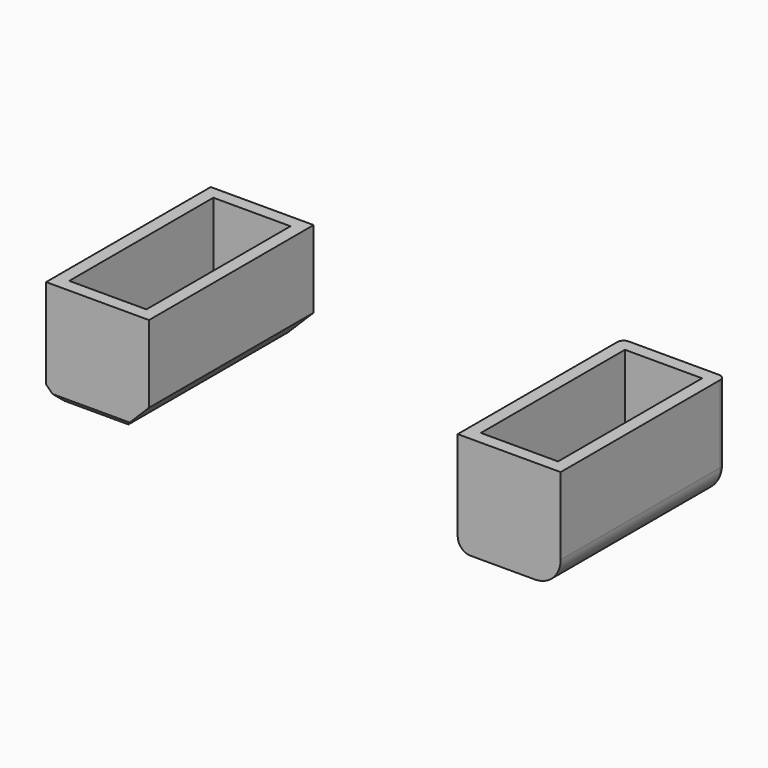
from build123d import *

# Parameters (mm, degrees)
F0_W     = 12.7
F0_H     = 25.4
F1_DEPTH = 12.7
F3_SIZE  = 3.175
F4_SIZE  = 1.5875
F5_SIZE  = 0.79375
F6_T     = -1.5875
F7_R     = 3.175
F8_R     = 1.5875
F9_R     = 0.79375
F10_T    = 1.5875


# Not quite as in the source:
# - a shell that OpenCascade refuses in one call is made with other operations: the cavity is built on its own and cut out


with BuildPart() as f1:
    # F0 (on Top) → F1 (new body)
    with BuildSketch(Plane.XY):
        with Locations((-17.8713803947, 23.258962822)):
            Rectangle(F0_W, F0_H)
    extrude(amount=F1_DEPTH)


with BuildPart() as f2_1:
    # F2: copy of F1
    add(f1.part.moved(Location((50.8, 0, 0))))

    # F7
    f7_edges = [f2_1.edges().sort_by_distance(p)[0] for p in [
        (39.27862, 23.258963, 0),
    ]]
    fillet(f7_edges, radius=F7_R)

    # F8
    f8_edges = [f2_1.edges().sort_by_distance(p)[0] for p in [
        (26.57862, 23.258963, 0),
    ]]
    fillet(f8_edges, radius=F8_R)

    # F9
    f9_edges = [f2_1.edges().sort_by_distance(p)[0] for p in [
        (32.13487, 35.958963, 0),
    ]]
    fillet(f9_edges, radius=F9_R)

    # F10: shell of thickness 1.5875, made by hand


with BuildPart() as f1_1:
    add(f1.part)

    # F3
    f3_edges = [f1_1.edges().sort_by_distance(p)[0] for p in [
        (-11.52138, 23.258963, 0),
    ]]
    chamfer(f3_edges, length=F3_SIZE)

    # F4
    f4_edges = [f1_1.edges().sort_by_distance(p)[0] for p in [
        (-24.22138, 23.258963, 0),
    ]]
    chamfer(f4_edges, length=F4_SIZE)

    # F5
    f5_edges = [f1_1.edges().sort_by_distance(p)[0] for p in [
        (-18.66513, 10.558963, 0),
    ]]
    chamfer(f5_edges, length=F5_SIZE)

    # F6
    f6_openings = [f1_1.faces().sort_by_distance(p)[0] for p in [
        (-17.87138, 23.258963, 12.7),
    ]]
    offset(amount=F6_T, openings=f6_openings)


with BuildPart() as f10_core1:
    # F10_t2: copy of F2_1
    add(f2_1.part)

    # the walls: a layer under each face that stays
    f10_faces = [f10_core1.faces().sort_by_distance(p)[0] for p in [
        (32.9286196053, 35.958962822, 6.746875),
        (39.2786196053, 22.862087822, 7.9375),
        (26.5786196053, 22.862087822, 7.14375),
        (32.9286196053, 10.558962822, 6.35),
        (38.3486836356, 22.862087822, 0.9299359697),
        (32.1348696053, 22.862087822, 0),
    ]]
    thicken(f10_faces, amount=-F10_T, mode=Mode.SUBTRACT)


with BuildPart() as f2_1_1:
    add(f2_1.part)

    # what is left inside the walls is the cavity
    f10_cavity = [f10_core1.part.solids().sort_by_distance(p)[0] for p in [
        (28.181995, 23.258963, 8.995833),
    ]]
    add(f10_cavity, mode=Mode.SUBTRACT)


solid = Compound([f1_1.part, f2_1_1.part])
